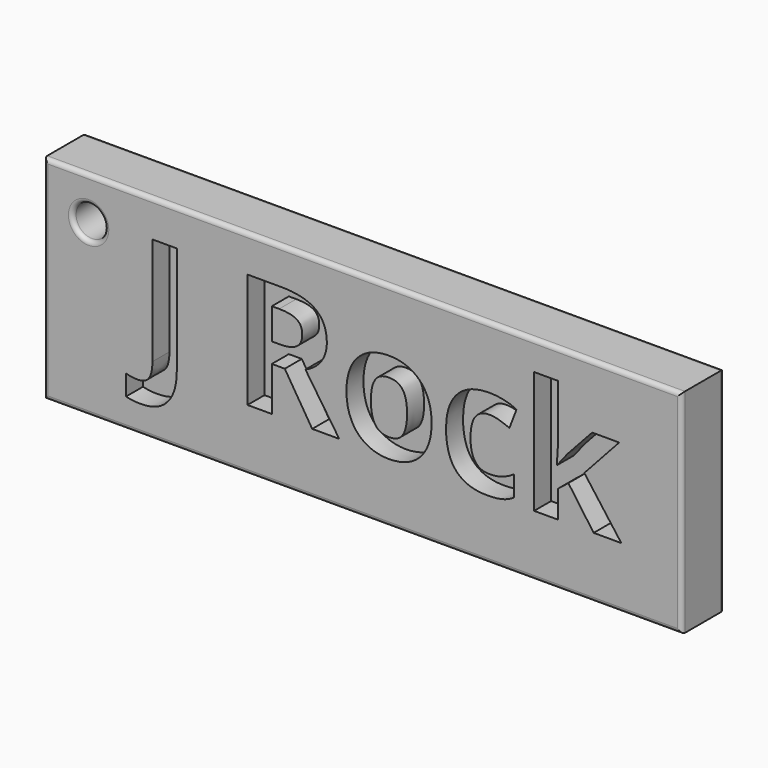
from build123d import *

# Parameters (mm, degrees)
F0_W         = 76.2
F0_H         = 25.4
F1_DEPTH     = 6.35
F2_R         = 1.905
F3_DEPTH     = 25.4
F4_R         = 0.508
F5_TEXT_SIZE = 19.2203326151
F6_DEPTH     = 2.54


# Not quite as in the source:
# - Text() gives the source's letters only with a copy of the font that has no kerning and outlines rounded to 1/6400 em; it was checked with that copy


with BuildPart() as f1:
    # F0 (on Front) → F1 (new body)
    with BuildSketch(Plane.XZ):
        Rectangle(F0_W, F0_H)
    extrude(amount=F1_DEPTH)

    # F2 (on face) → F3 (cut)
    with BuildSketch(Plane.XZ.offset(6.35)):
        with Locations((-32.7522344887, 7.6349042356)):
            Circle(F2_R)
    extrude(amount=-F3_DEPTH, mode=Mode.SUBTRACT)

    # F4
    f4_edges = [f1.edges().sort_by_distance(p)[0] for p in [
        (0, -6.35, 12.7),
        (38.1, -6.35, 0),
        (-38.1, -6.35, 0),
        (0, -6.35, -12.7),
        (-34.657234, -6.35, 7.634904),
        (-34.657234, 0, 7.634904),
        (0, 0, 12.7),
        (-38.1, 0, 0),
        (0, 0, -12.7),
        (38.1, 0, 0),
    ]]
    fillet(f4_edges, radius=F4_R)

    # F5 (on face) → F6 (cut)
    with BuildSketch(Plane.XZ.offset(6.35)):
        with Locations((-26.8561418634, -5.3944545798)):
            Text('J Rock', F5_TEXT_SIZE, font='Open Sans', font_style=FontStyle.BOLD, text_align=(TextAlign.LEFT, TextAlign.BOTTOM))
    extrude(amount=-F6_DEPTH, mode=Mode.SUBTRACT)


solid = f1.part
